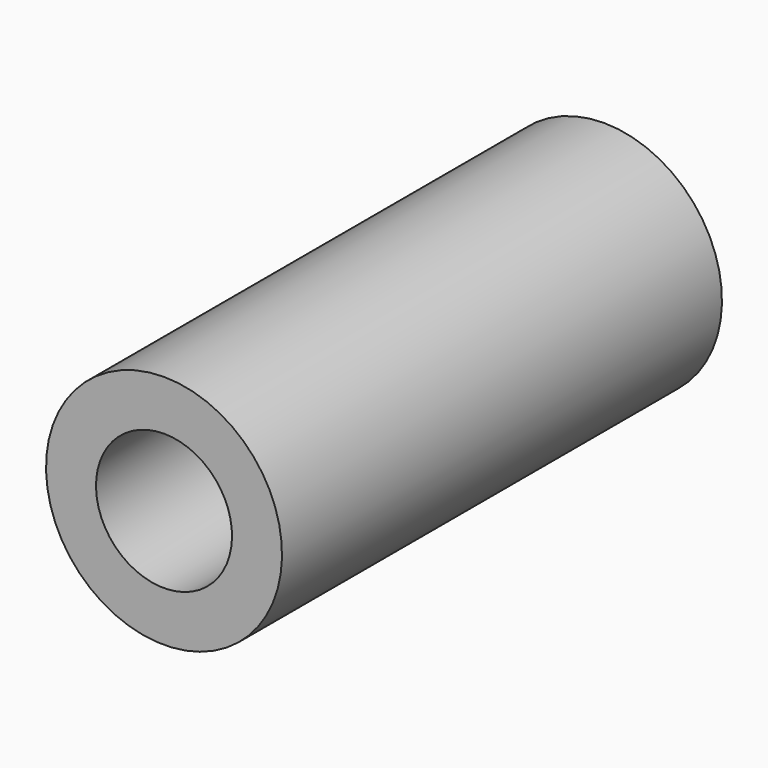
from build123d import *

# Parameters (mm, degrees)
F2_SIZE = 0.09999


# Not quite as in the source:
# - a fillet or chamfer is up to 0.001 mm smaller than in the source, because OpenCascade refuses the exact size


with BuildPart() as f1:
    # F0 (on Right) → F1 (revolve)
    with BuildSketch(Plane.YZ):
        with BuildLine():
            ThreePointArc((7.5617104388, 2.8), (8.3591026496, 4.0638625595), (9.425, 5.1112620751))
            Line((9.425, 5.1112620751), (9.425, 5.9))
            Line((9.425, 5.9), (-18.075, 5.9))
            Line((-18.075, 5.9), (-18.075, 3.4))
            Line((-18.075, 3.4), (-7.075, 3.4))
            Line((-7.075, 3.4), (-7.075, 3.3))
            Line((-7.075, 3.3), (-6.425, 3.3))
            Line((-6.425, 3.3), (6.425, 3.3))
            Line((6.425, 3.3), (6.925, 3.3))
            Line((6.925, 3.3), (6.925, 2.8))
            Line((6.925, 2.8), (7.5617104388, 2.8))
        make_face()
        Polygon((6.425, 3.3), (6.925, 2.8), (6.925, 3.3), align=None)
    revolve(axis=Axis((0, 2.1126118954, 0), (0, 1, 0)))

    # F2 (size 0.1 in the source; OpenCascade refuses exactly that, so slightly less here)
    f2_edges = [f1.edges().sort_by_distance(p)[0] for p in [
        (0, -7.075, -3.4),
    ]]
    chamfer(f2_edges, length=F2_SIZE)


solid = f1.part
